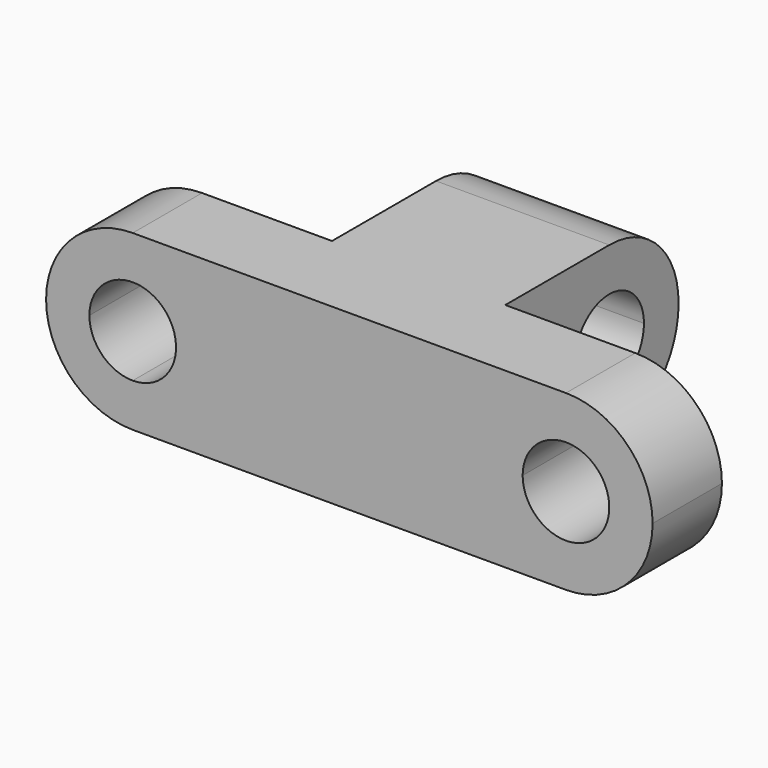
from build123d import *

# Parameters (mm, degrees)
F0_W     = 31.75
F0_H     = 12.7
F1_DEPTH = 25.4
F3_DEPTH = 25.4
F5_DEPTH = 25.4
F7_DEPTH = 25.4
F8_R     = 12.69999


# Not quite as in the source:
# - a fillet or chamfer is up to 0.001 mm smaller than in the source, because OpenCascade refuses the exact size


with BuildPart() as f1:
    # F0 (on Top) → F1 (new body)
    with BuildSketch(Plane.XY):
        Polygon((0, 12.7), (0, 0), (25.4, 0), (25.4, 12.7), (25.4, 44.45), (0, 44.45), align=None)
        with Locations((-15.875, 6.35)):
            Rectangle(F0_W, F0_H)
        with Locations((41.275, 6.35)):
            Rectangle(F0_W, F0_H)
    extrude(amount=F1_DEPTH)

    # F2 (on face) → F3 (cut)
    with BuildSketch(Plane.YZ.offset(25.4)):
        with BuildLine():
            ThreePointArc((38.1, 12.7), (36.2401280605, 17.1901280605), (31.75, 19.05))
            ThreePointArc((31.75, 19.05), (27.2598719395, 8.2098719395), (38.1, 12.7))
        make_face()
    extrude(amount=-F3_DEPTH, mode=Mode.SUBTRACT)

    # F4 (on face) → F5 (cut)
    with BuildSketch(Plane(origin=(0, 12.7, 0), x_dir=(-1, 0, 0), z_dir=(0, 1, 0))):
        with BuildLine():
            ThreePointArc((-44.45, 19.05), (-48.9401280605, 8.2098719395), (-38.1, 12.7))
            ThreePointArc((-38.1, 12.7), (-39.9598719395, 17.1901280605), (-44.45, 19.05))
        make_face()
    extrude(amount=-F5_DEPTH, mode=Mode.SUBTRACT)

    # F6 (on face) → F7 (cut)
    with BuildSketch(Plane(origin=(0, 12.7, 0), x_dir=(-1, 0, 0), z_dir=(0, 1, 0))):
        with BuildLine():
            ThreePointArc((19.05, 6.35), (23.5401280605, 8.2098719395), (25.4, 12.7))
            ThreePointArc((25.4, 12.7), (14.5598719395, 17.1901280605), (19.05, 6.35))
        make_face()
    extrude(amount=-F7_DEPTH, mode=Mode.SUBTRACT)

    # F8 (radius 12.7 in the source; OpenCascade refuses exactly that, so slightly less here)
    f8_edges = [f1.edges().sort_by_distance(p)[0] for p in [
        (57.15, 6.35, 25.4),
        (57.15, 6.35, 0),
        (12.7, 44.45, 25.4),
        (12.7, 44.45, 0),
        (-31.75, 6.35, 0),
        (-31.75, 6.35, 25.4),
    ]]
    fillet(f8_edges, radius=F8_R)


solid = f1.part
